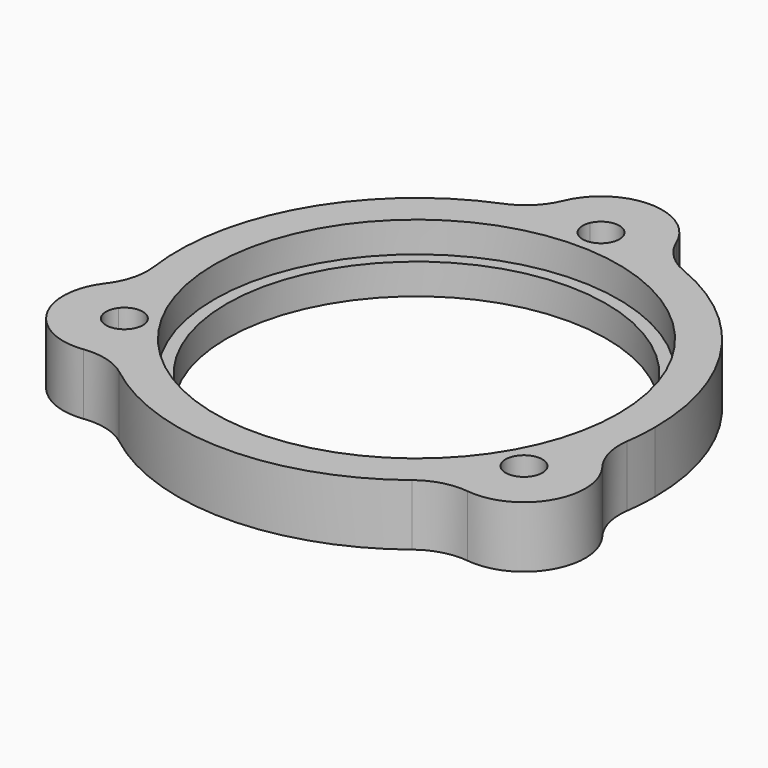
from build123d import *

# Parameters (mm, degrees)
F0_R     = 20.955
F0_R_2   = 19.685
F1_DEPTH = 3.175
F2_DEPTH = 6.35
F3_R     = 6.35


with BuildPart() as f1:
    # F0 (on Top) → F1 (new body)
    with BuildSketch(Plane.XY):
        Circle(F0_R)
        Circle(F0_R_2, mode=Mode.SUBTRACT)
    extrude(amount=F1_DEPTH)

    # F0 (on Top) → F2 (join)
    with BuildSketch(Plane.XY):
        with BuildLine():
            ThreePointArc((23.9050999455, -6.4692674698), (24.5490837421, -3.2630832697), (24.765, 0))
            ThreePointArc((24.765, 0), (19.6285885254, 15.1004548773), (6.35, 23.9370575677))
            ThreePointArc((6.35, 23.9370575677), (4.0651088886, 24.4290833787), (1.7440091422, 24.703515076))
            ThreePointArc((1.7440091422, 24.703515076), (1.8643178935, 24.3286489263), (1.905, 23.9370575677))
            ThreePointArc((1.905, 23.9370575677), (-0.3915913586, 22.0727396742), (-1.7440091422, 24.703515076))
            ThreePointArc((-1.7440091422, 24.703515076), (-4.0651088886, 24.4290833787), (-6.35, 23.9370575677))
            ThreePointArc((-6.35, 23.9370575677), (-21.4471191247, 12.3825), (-23.9050999455, -6.4692674698))
            ThreePointArc((-23.9050999455, -6.4692674698), (-23.1887612414, -8.6940541227), (-22.2658761897, -10.8414013165))
            ThreePointArc((-22.2658761897, -10.8414013165), (-20.1370690632, -10.1581864481), (-18.8250999455, -11.9685287839))
            ThreePointArc((-18.8250999455, -11.9685287839), (-19.3113489683, -13.239815795), (-20.5218670475, -13.8621137596))
            ThreePointArc((-20.5218670475, -13.8621137596), (-19.1236523528, -15.735029256), (-17.5550999455, -17.4677900979))
            ThreePointArc((-17.5550999455, -17.4677900979), (0, -24.765), (17.5550999455, -17.4677900979))
            ThreePointArc((17.5550999455, -17.4677900979), (19.1236523528, -15.735029256), (20.5218670475, -13.8621137596))
            ThreePointArc((20.5218670475, -13.8621137596), (19.0803215513, -11.0160287839), (22.2658761897, -10.8414013165))
            ThreePointArc((22.2658761897, -10.8414013165), (23.1887612414, -8.6940541227), (23.9050999455, -6.4692674698))
        make_face()
        Circle(F0_R, mode=Mode.SUBTRACT)
        with BuildLine():
            ThreePointArc((1.7440091422, 24.703515076), (4.0651088886, 24.4290833787), (6.35, 23.9370575677))
            ThreePointArc((6.35, 23.9370575677), (0, 30.2870575677), (-6.35, 23.9370575677))
            ThreePointArc((-6.35, 23.9370575677), (-4.0651088886, 24.4290833787), (-1.7440091422, 24.703515076))
            ThreePointArc((-1.7440091422, 24.703515076), (0, 25.8420575677), (1.7440091422, 24.703515076))
        make_face()
        with BuildLine():
            ThreePointArc((17.5550999455, -17.4677900979), (26.2293612595, -15.1435287839), (23.9050999455, -6.4692674698))
            ThreePointArc((23.9050999455, -6.4692674698), (23.1887612414, -8.6940541227), (22.2658761897, -10.8414013165))
            ThreePointArc((22.2658761897, -10.8414013165), (22.5404422812, -11.3754979015), (22.6350999455, -11.9685287839))
            ThreePointArc((22.6350999455, -11.9685287839), (22.0013869566, -13.3872797611), (20.5218670475, -13.8621137596))
            ThreePointArc((20.5218670475, -13.8621137596), (19.1236523528, -15.735029256), (17.5550999455, -17.4677900979))
        make_face()
        with BuildLine():
            ThreePointArc((-22.2658761897, -10.8414013165), (-23.1887612414, -8.6940541227), (-23.9050999455, -6.4692674698))
            ThreePointArc((-23.9050999455, -6.4692674698), (-26.2293612595, -15.1435287839), (-17.5550999455, -17.4677900979))
            ThreePointArc((-17.5550999455, -17.4677900979), (-19.1236523528, -15.735029256), (-20.5218670475, -13.8621137596))
            ThreePointArc((-20.5218670475, -13.8621137596), (-22.3798783397, -12.9210287839), (-22.2658761897, -10.8414013165))
        make_face()
    extrude(amount=F2_DEPTH)

    # F3
    f3_edges = [f1.edges().sort_by_distance(p)[0] for p in [
        (6.35, 23.937058, 3.175),
        (-23.9051, -6.469267, 3.175),
        (17.5551, -17.46779, 3.175),
        (23.9051, -6.469267, 3.175),
        (-6.35, 23.937058, 3.175),
        (-17.5551, -17.46779, 3.175),
    ]]
    fillet(f3_edges, radius=F3_R)


solid = f1.part
